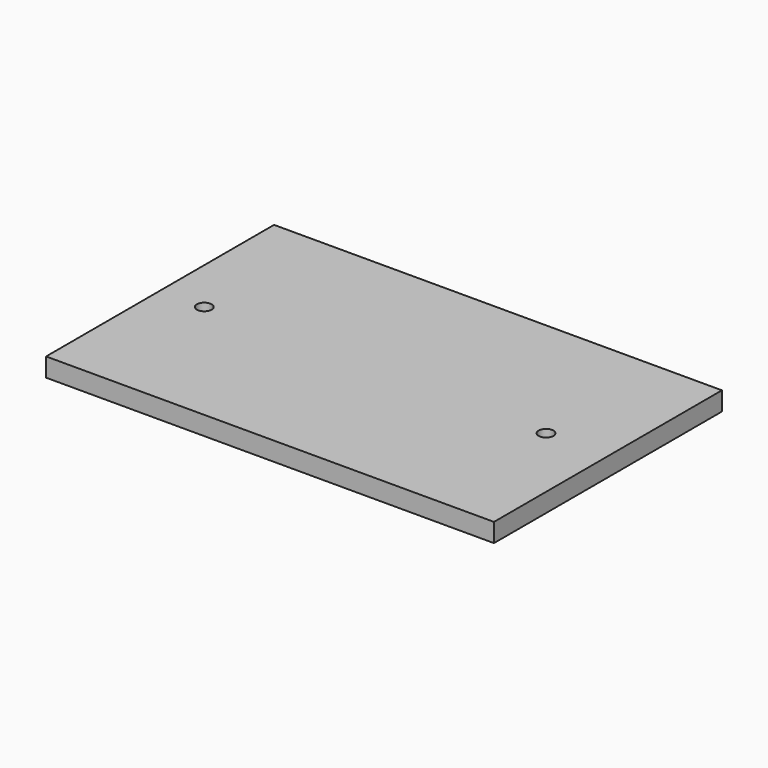
from build123d import *

# Parameters (mm, degrees)
F0_W     = 76
F0_H     = 48.35
F0_R     = 1.25
F1_DEPTH = 3.175


# Not quite as in the source:
# - a length typed as a fraction of an inch, garbled in the dataset ("3 / 203.2 mm" for 3/8 in), is restored
# - a feature names something its author has since deleted; it is built from what else it names


with BuildPart() as f1:
    # F0 (on Top) → F1 (new body)
    with BuildSketch(Plane.XY):
        with Locations((20.4403014183, -5.2875590026)):
            Rectangle(F0_W, F0_H)
        with Locations((-10.0596985817, -5.2875590026)):
            Circle(F0_R, mode=Mode.SUBTRACT)
        with Locations((47.9403014183, -5.2875590026)):
            Circle(F0_R, mode=Mode.SUBTRACT)
    extrude(amount=F1_DEPTH)


solid = f1.part
